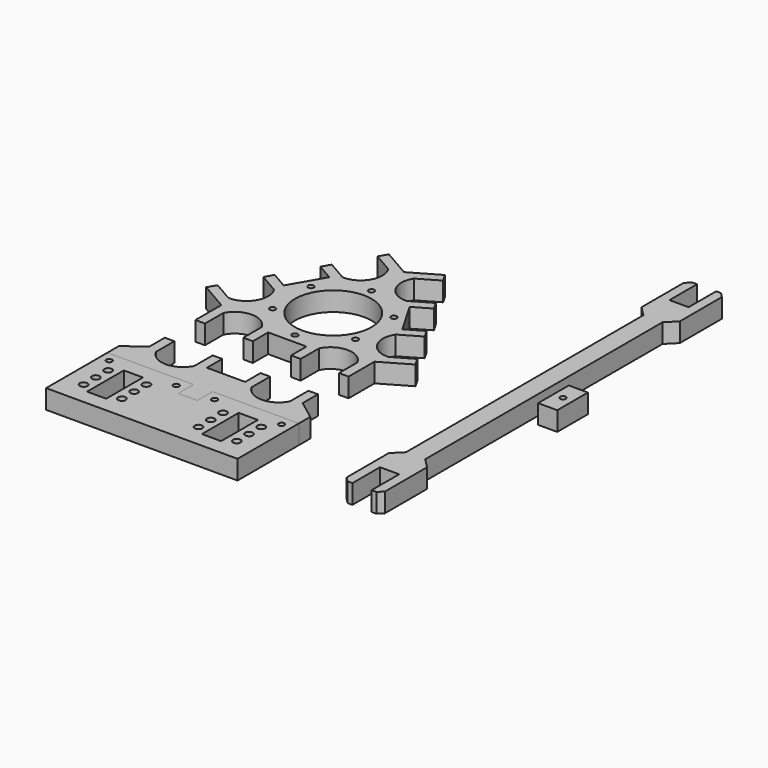
from build123d import *

# Parameters (mm, degrees)
F0_R     = 1.5
F0_R_2   = 20
F1_DEPTH = 10
F0_R_3   = 2
F0_W     = 10
F0_H     = 24
F0_H_2   = 20
F2_DEPTH = 10


# Not quite as in the source:
# - a feature names something its author has since deleted; it is built from what else it names


with BuildPart() as f1:
    # F0 (on Top) → F1 (new body)
    with BuildSketch(Plane.XY):
        with BuildLine():
            Line((-10, -30), (0, -30))
            Line((0, -30), (10, -30))
            Line((10, -30), (10, -40))
            Line((10, -40), (15, -40))
            Line((15, -40), (15, -28))
            ThreePointArc((15, -28), (25, -21.903882032), (35, -28))
            Line((35, -28), (35, -40))
            Line((35, -40), (40, -40))
            Line((40, -40), (40, -23.0940107676))
            Line((40, -23.0940107676), (54.6410161514, -14.6410161514))
            Line((54.6410161514, -14.6410161514), (52.1410161514, -10.3108891325))
            Line((52.1410161514, -10.3108891325), (41.748711306, -16.3108891325))
            ThreePointArc((41.748711306, -16.3108891325), (31.4693182812, -10.6986940786), (31.748711306, 1.0096189432))
            Line((31.748711306, 1.0096189432), (42.1410161514, 7.0096189432))
            Line((42.1410161514, 7.0096189432), (39.6410161514, 11.3397459622))
            Line((39.6410161514, 11.3397459622), (30.9807621135, 6.3397459622))
            Line((30.9807621135, 6.3397459622), (25.9807621135, 15))
            Line((25.9807621135, 15), (20.9807621135, 23.6602540378))
            Line((20.9807621135, 23.6602540378), (29.6410161514, 28.6602540378))
            Line((29.6410161514, 28.6602540378), (27.1410161514, 32.9903810568))
            Line((27.1410161514, 32.9903810568), (16.748711306, 26.9903810568))
            ThreePointArc((16.748711306, 26.9903810568), (6.4693182812, 32.6025761106), (6.748711306, 44.3108891325))
            Line((6.748711306, 44.3108891325), (17.1410161514, 50.3108891325))
            Line((17.1410161514, 50.3108891325), (14.6410161514, 54.6410161514))
            Line((14.6410161514, 54.6410161514), (0, 46.1880215352))
            Line((0, 46.1880215352), (-14.6410161514, 54.6410161514))
            Line((-14.6410161514, 54.6410161514), (-17.1410161514, 50.3108891325))
            Line((-17.1410161514, 50.3108891325), (-6.748711306, 44.3108891325))
            ThreePointArc((-6.748711306, 44.3108891325), (-6.4693182812, 32.6025761106), (-16.748711306, 26.9903810568))
            Line((-16.748711306, 26.9903810568), (-27.1410161514, 32.9903810568))
            Line((-27.1410161514, 32.9903810568), (-29.6410161514, 28.6602540378))
            Line((-29.6410161514, 28.6602540378), (-20.9807621135, 23.6602540378))
            Line((-20.9807621135, 23.6602540378), (-25.9807621135, 15))
            Line((-25.9807621135, 15), (-30.9807621135, 6.3397459622))
            Line((-30.9807621135, 6.3397459622), (-39.6410161514, 11.3397459622))
            Line((-39.6410161514, 11.3397459622), (-42.1410161514, 7.0096189432))
            Line((-42.1410161514, 7.0096189432), (-31.748711306, 1.0096189432))
            ThreePointArc((-31.748711306, 1.0096189432), (-31.4693182812, -10.6986940786), (-41.748711306, -16.3108891325))
            Line((-41.748711306, -16.3108891325), (-52.1410161514, -10.3108891325))
            Line((-52.1410161514, -10.3108891325), (-54.6410161514, -14.6410161514))
            Line((-54.6410161514, -14.6410161514), (-40, -23.0940107676))
            Line((-40, -23.0940107676), (-40, -40))
            Line((-40, -40), (-35, -40))
            Line((-35, -40), (-35, -28))
            ThreePointArc((-35, -28), (-25, -21.903882032), (-15, -28))
            Line((-15, -28), (-15, -40))
            Line((-15, -40), (-10, -40))
            Line((-10, -40), (-10, -30))
        make_face()
        with Locations((-21.6506350946, -12.5)):
            Circle(F0_R, mode=Mode.SUBTRACT)
        with Locations((0, -25)):
            Circle(F0_R, mode=Mode.SUBTRACT)
        with Locations((21.6506350946, -12.5)):
            Circle(F0_R, mode=Mode.SUBTRACT)
        with Locations((-21.6506350946, 12.5)):
            Circle(F0_R, mode=Mode.SUBTRACT)
        Circle(F0_R_2, mode=Mode.SUBTRACT)
        with Locations((21.6506350946, 12.5)):
            Circle(F0_R, mode=Mode.SUBTRACT)
        with Locations((0, 25)):
            Circle(F0_R, mode=Mode.SUBTRACT)
    extrude(amount=F1_DEPTH)


with BuildPart() as f1b:
    # F0 (on Top) → F1, piece 2 (new body)
    with BuildSketch(Plane.XY):
        Polygon((-5, -85), (-50, -85), (-50, -125), (50, -125), (50, -85), (5, -85), (5, -95), (0, -95), (-5, -95), align=None)
        with Locations((-40, -113)):
            Circle(F0_R_3, mode=Mode.SUBTRACT)
        with Locations((-40, -105)):
            Circle(F0_R_3, mode=Mode.SUBTRACT)
        with Locations((-40, -97)):
            Circle(F0_R_3, mode=Mode.SUBTRACT)
        with Locations((-20, -113)):
            Circle(F0_R_3, mode=Mode.SUBTRACT)
        with Locations((-30, -105)):
            Rectangle(F0_W, F0_H, mode=Mode.SUBTRACT)
        with Locations((-20, -105)):
            Circle(F0_R_3, mode=Mode.SUBTRACT)
        with Locations((-20, -97)):
            Circle(F0_R_3, mode=Mode.SUBTRACT)
        with Locations((-45, -90)):
            Circle(F0_R, mode=Mode.SUBTRACT)
        with Locations((-10, -90)):
            Circle(F0_R, mode=Mode.SUBTRACT)
        with Locations((20, -113)):
            Circle(F0_R_3, mode=Mode.SUBTRACT)
        with Locations((20, -105)):
            Circle(F0_R_3, mode=Mode.SUBTRACT)
        with Locations((20, -97)):
            Circle(F0_R_3, mode=Mode.SUBTRACT)
        with Locations((30, -105)):
            Rectangle(F0_W, F0_H, mode=Mode.SUBTRACT)
        with Locations((10, -90)):
            Circle(F0_R, mode=Mode.SUBTRACT)
        with Locations((40, -113)):
            Circle(F0_R_3, mode=Mode.SUBTRACT)
        with Locations((40, -105)):
            Circle(F0_R_3, mode=Mode.SUBTRACT)
        with Locations((40, -97)):
            Circle(F0_R_3, mode=Mode.SUBTRACT)
        with Locations((45, -90)):
            Circle(F0_R, mode=Mode.SUBTRACT)
    extrude(amount=F1_DEPTH)


with BuildPart() as f1c:
    # F0 (on Top) → F1, piece 3 (new body)
    with BuildSketch(Plane.XY):
        Polygon((100, 77.5), (100, 0), (100, -77.5), (95, -82.5), (95, -110), (97.5, -112.5), (100, -112.5), (100, -94.5), (110, -94.5), (110, -112.5), (112.5, -112.5), (115, -110), (115, -82.5), (110, -77.5), (110, 0), (110, 77.5), (115, 82.5), (115, 110), (112.5, 112.5), (110, 112.5), (110, 94.5), (100, 94.5), (100, 112.5), (97.5, 112.5), (95, 110), (95, 82.5), align=None)
    extrude(amount=F1_DEPTH)


with BuildPart() as f1d:
    # F0 (on Top) → F1, piece 4 (new body)
    with BuildSketch(Plane.XY):
        with Locations((120, 0)):
            Rectangle(F0_W, F0_H_2)
        with Locations((120, 0)):
            Circle(F0_R, mode=Mode.SUBTRACT)
    extrude(amount=F1_DEPTH)


with BuildPart() as f2:
    # F0 (on Top) → F2 (new body)
    with BuildSketch(Plane.XY):
        with BuildLine():
            Line((-35, -60), (-40, -60))
            Line((-40, -60), (-40, -70))
            Line((-40, -70), (-50, -77.5))
            Line((-50, -77.5), (-50, -85))
            Line((-50, -85), (-5, -85))
            Line((-5, -85), (-5, -95))
            Line((-5, -95), (0, -95))
            Line((0, -95), (5, -95))
            Line((5, -95), (5, -85))
            Line((5, -85), (50, -85))
            Line((50, -85), (50, -77.5))
            Line((50, -77.5), (40, -70))
            Line((40, -70), (40, -60))
            Line((40, -60), (35, -60))
            Line((35, -60), (35, -72))
            ThreePointArc((35, -72), (25, -78.096117968), (15, -72))
            Line((15, -72), (15, -60))
            Line((15, -60), (10, -60))
            Line((10, -60), (10, -70))
            Line((10, -70), (0, -70))
            Line((0, -70), (-10, -70))
            Line((-10, -70), (-10, -60))
            Line((-10, -60), (-15, -60))
            Line((-15, -60), (-15, -72))
            ThreePointArc((-15, -72), (-25, -78.096117968), (-35, -72))
            Line((-35, -72), (-35, -60))
        make_face()
    extrude(amount=F2_DEPTH)


solid = Compound([f1.part, f1b.part, f1c.part, f1d.part, f2.part])
